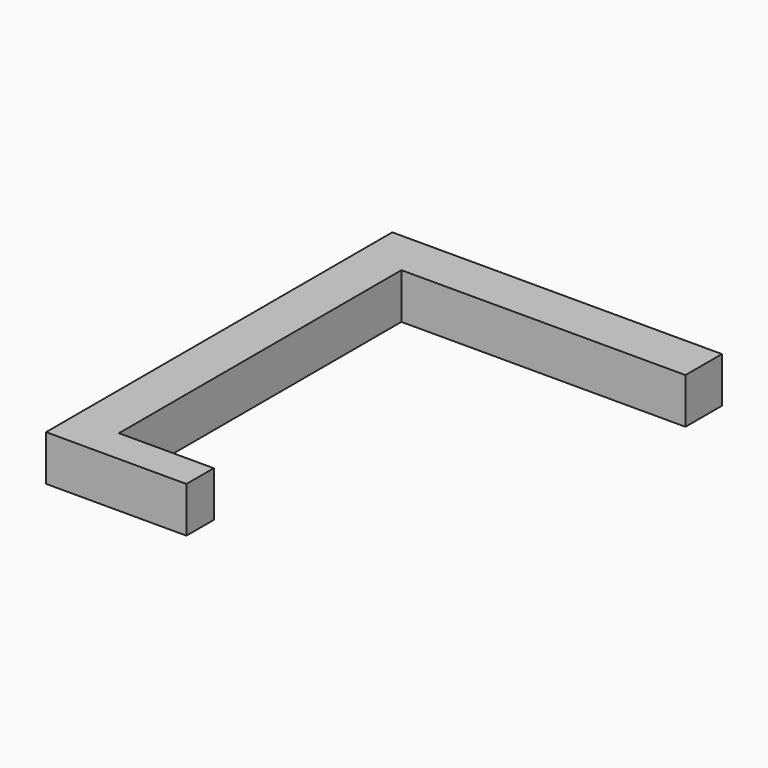
from build123d import *

# Parameters (mm, degrees)
F0_W     = 24.9417738095
F0_H     = 4
F0_W_2   = 8.3235937208
F0_H_2   = 3
F1_DEPTH = 4


# Not quite as in the source:
# - the program builds the solid bodies; features that only make, move or delete a surface that nothing else refers to are left out


with BuildPart() as f1:
    # F0 (on Top) → F1 (new body)
    with BuildSketch(Plane.XY):
        Polygon((-19.8069426268, 31.5581213795), (-23.8069426268, 31.5581213795), (-23.8069426268, -6.4418786205), (-19.8069426268, -6.4418786205), (-19.8069426268, -3.4418786205), (-19.8069426268, 27.5581213795), align=None)
        with Locations((-7.3360557221, 29.5581213795)):
            Rectangle(F0_W, F0_H)
        with Locations((-15.6451457664, -4.9418786205)):
            Rectangle(F0_W_2, F0_H_2)
    extrude(amount=F1_DEPTH)


solid = f1.part
